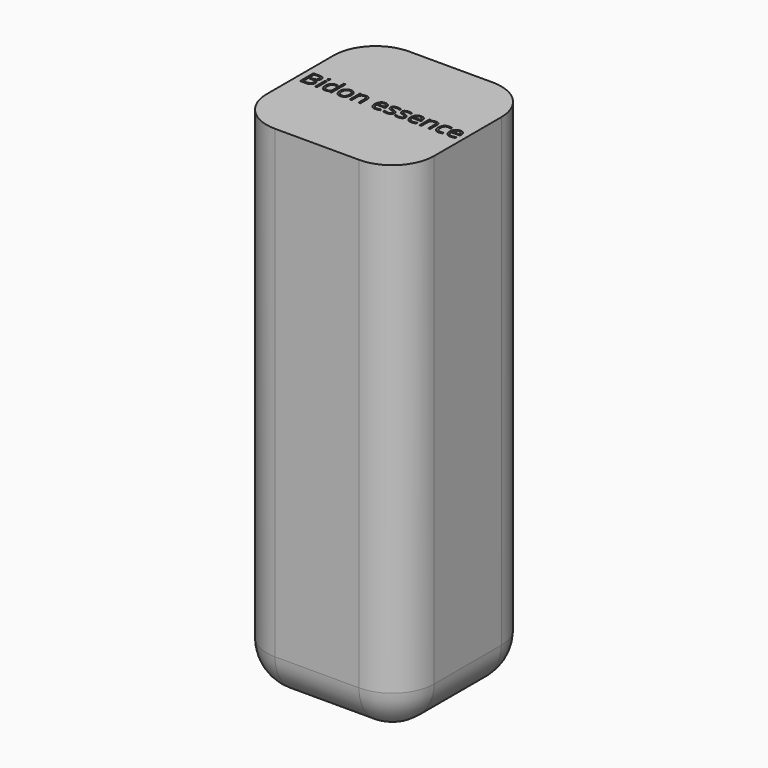
from build123d import *

# Parameters (mm, degrees)
F0_W         = 200.66
F0_H         = 200.66
F1_DEPTH     = 607.06
F2_TEXT_SIZE = 28.3252628891
F3_DEPTH     = 5
F4_R         = 50


# Not quite as in the source:
# - Text() gives the source's letters only with a copy of the font that has no kerning and outlines rounded to 1/6400 em; it was checked with that copy


with BuildPart() as f1:
    # F0 (on Top) → F1 (new body)
    with BuildSketch(Plane.XY):
        Rectangle(F0_W, F0_H)
    extrude(amount=F1_DEPTH)

    # F2 (on face) → F3 (cut)
    with BuildSketch(Plane.XY.offset(607.06)):
        with Locations((-95.33, -10.1970946401)):
            Text('Bidon essence', F2_TEXT_SIZE, font='Open Sans', text_align=(TextAlign.LEFT, TextAlign.BOTTOM))
    extrude(amount=-F3_DEPTH, mode=Mode.SUBTRACT)

    # F4
    f4_edges = [f1.edges().sort_by_distance(p)[0] for p in [
        (100.33, -100.33, 303.53),
        (100.33, 100.33, 303.53),
        (-100.33, -100.33, 303.53),
        (-100.33, 100.33, 303.53),
        (0, -100.33, 0),
        (100.33, 0, 0),
        (0, 100.33, 0),
        (-100.33, 0, 0),
    ]]
    fillet(f4_edges, radius=F4_R)


solid = f1.part
